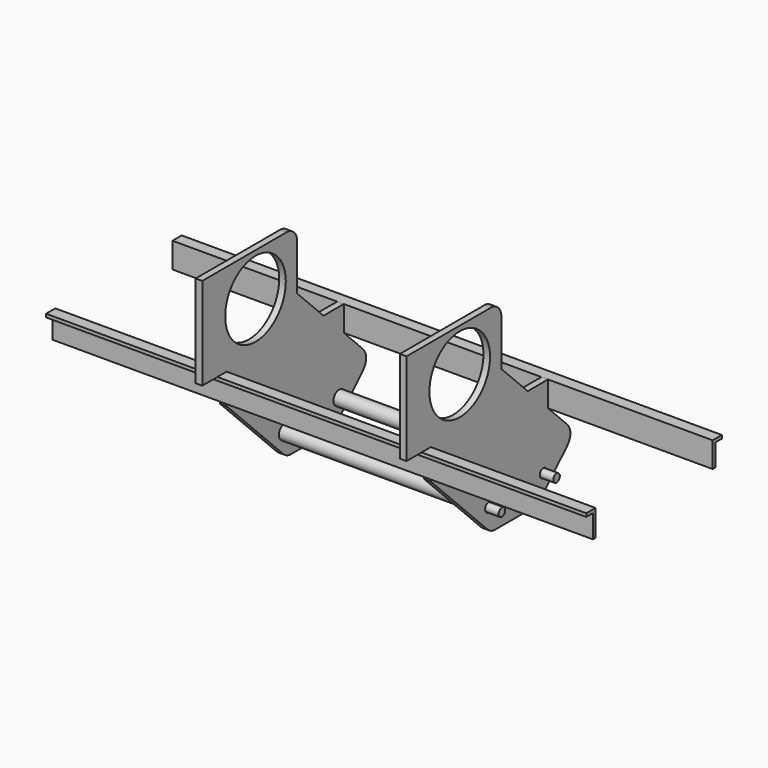
from build123d import *

# Parameters (mm, degrees)
F4_DEPTH      = 260.35
F4_DEPTH_BACK = 260.35
F2_R          = 6.858
F2_R_2        = 4.3688
F5_DEPTH      = 95.25
F5_DEPTH_BACK = 95.25
F2_R_3        = 3.96875
F6_DEPTH      = 114.3
F6_DEPTH_BACK = 114.3
F7_R          = 4.3688
F7_R_2        = 6.858
F7_R_3        = 36.5125
F8_DEPTH      = 6.35


# Not quite as in the source:
# - a variable given as a bare number and used for a length is read in inches; the dataset says mm whatever the document's units were


with BuildPart() as f4:
    # F2 (on Right) → F4 (new body, two sides)
    with BuildSketch(Plane.YZ) as f4_sk:
        Polygon((29.3066704261, -88.9), (18.1941704261, -88.9), (18.1941704261, -92.075), (26.1316704261, -92.075), (26.1316704261, -114.3), (29.3066704261, -114.3), align=None)
    extrude(amount=F4_DEPTH)
    extrude(f4_sk.sketch, amount=-F4_DEPTH_BACK)


with BuildPart() as f4b:
    # F2 (on Right) → F4, piece 2 (new body, two sides)
    with BuildSketch(Plane.YZ) as f4_2_sk:
        Polygon((181.6048598051, -88.9), (170.4923598051, -88.9), (170.4923598051, -113.3423598051), (173.6673598051, -113.3423598051), (173.6673598051, -92.075), (181.6048598051, -92.075), align=None)
    extrude(amount=F4_DEPTH)
    extrude(f4_2_sk.sketch, amount=-F4_DEPTH_BACK)


with BuildPart() as f5:
    # F2 (on Right) → F5 (new body, two sides)
    with BuildSketch(Plane.YZ) as f5_sk:
        with Locations((164.9153412521, -166.1370060391)):
            Circle(F2_R)
        with Locations((164.9153412521, -166.1370060391)):
            Circle(F2_R_2, mode=Mode.SUBTRACT)
    extrude(amount=F5_DEPTH)
    extrude(f5_sk.sketch, amount=-F5_DEPTH_BACK)


with BuildPart() as f5b:
    # F2 (on Right) → F5, piece 2 (new body, two sides)
    with BuildSketch(Plane.YZ) as f5_2_sk:
        with Locations((99.0900638847, -168.3820700693)):
            Circle(F2_R)
        with Locations((99.0900638847, -168.3820700693)):
            Circle(F2_R_2, mode=Mode.SUBTRACT)
    extrude(amount=F5_DEPTH)
    extrude(f5_2_sk.sketch, amount=-F5_DEPTH_BACK)


with BuildPart() as f6:
    # F2 (on Right) → F6 (new body, two sides)
    with BuildSketch(Plane.YZ) as f6_sk:
        with Locations((99.0900638847, -168.3820700693)):
            Circle(F2_R_3)
    extrude(amount=F6_DEPTH)
    extrude(f6_sk.sketch, amount=-F6_DEPTH_BACK)


with BuildPart() as f6b:
    # F2 (on Right) → F6, piece 2 (new body, two sides)
    with BuildSketch(Plane.YZ) as f6_2_sk:
        with Locations((164.9153412521, -166.1370060391)):
            Circle(F2_R_3)
    extrude(amount=F6_DEPTH)
    extrude(f6_2_sk.sketch, amount=-F6_DEPTH_BACK)


with BuildPart() as f8:
    # F7 (on face) → F8 (new body)
    with BuildSketch(Plane.YZ.offset(95.25)):
        with BuildLine():
            ThreePointArc((97.8537562482, -186.7537562482), (101.9739327783, -189.5067701901), (106.8340123693, -190.4735001272))
            Line((106.8340123693, -190.4735001272), (152.5604266743, -190.4735001272))
            ThreePointArc((152.5604266743, -190.4735001272), (157.4205062654, -189.5067701901), (161.5406827954, -186.7537562482))
            Line((161.5406827954, -186.7537562482), (193.7419634008, -154.5524756429))
            ThreePointArc((193.7419634008, -154.5524756429), (197.4617072797, -145.5722195218), (193.7419634008, -136.5919634008))
            Line((193.7419634008, -136.5919634008), (170.4923598051, -113.3423598051))
            Line((170.4923598051, -113.3423598051), (170.4923598051, -88.9))
            Line((170.4923598051, -88.9), (146.05, -88.9))
            Line((146.05, -88.9), (114.3, -57.15))
            Line((114.3, -57.15), (114.3, -12.7))
            ThreePointArc((114.3, -12.7), (110.5802561211, -3.7197438789), (101.6, 0))
            Line((101.6, 0), (0, 0))
            Line((0, 0), (0, -88.9))
            Line((0, -88.9), (29.3066704261, -88.9))
            Line((29.3066704261, -88.9), (29.3066704261, -118.2066704261))
            Line((29.3066704261, -118.2066704261), (97.8537562482, -186.7537562482))
        make_face()
        with Locations((99.0900638847, -168.3820700693)):
            Circle(F7_R, mode=Mode.SUBTRACT)
        with Locations((164.9153412521, -166.1370060391)):
            Circle(F7_R_2, mode=Mode.SUBTRACT)
        with Locations((64.14262, -41.275)):
            Circle(F7_R_3, mode=Mode.SUBTRACT)
        with Locations((164.9153412521, -166.1370060391)):
            Circle(F7_R_2)
        with Locations((164.9153412521, -166.1370060391)):
            Circle(F7_R, mode=Mode.SUBTRACT)
    extrude(amount=F8_DEPTH)


with BuildPart() as f9_1:
    # F9: instance of F8
    add(f8.part.mirror(Plane.YZ))


solid = Compound([f4.part, f4b.part, f5.part, f5b.part, f6.part, f6b.part, f8.part, f9_1.part])
